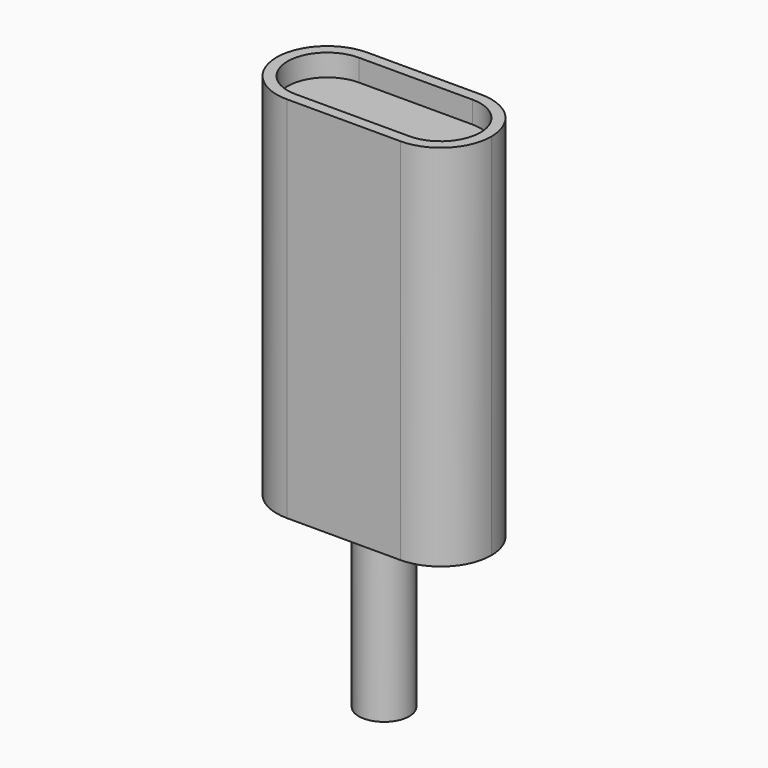
from build123d import *

# Parameters (mm, degrees)
F0_W     = 12.75
F0_H     = 6
F1_DEPTH = 21.9
F2_R     = 2.99999
F3_R     = 1.5
F4_DEPTH = 10
F6_DEPTH = 1.3


# Not quite as in the source:
# - a fillet or chamfer is up to 0.001 mm smaller than in the source, because OpenCascade refuses the exact size


with BuildPart() as f1:
    # F0 (on Top) → F1 (new body)
    with BuildSketch(Plane.XY):
        Rectangle(F0_W, F0_H)
    extrude(amount=F1_DEPTH)

    # F2 (radius 3 in the source; OpenCascade refuses exactly that, so slightly less here)
    f2_edges = [f1.edges().sort_by_distance(p)[0] for p in [
        (-6.375, -3, 10.95),
        (-6.375, 3, 10.95),
        (6.375, -3, 10.95),
        (6.375, 3, 10.95),
    ]]
    fillet(f2_edges, radius=F2_R)

    # F3 (on face) → F4 (join)
    with BuildSketch(Plane(origin=(0, 0, 0), x_dir=(1, 0, 0), z_dir=(0, 0, -1))):
        Circle(F3_R)
    extrude(amount=F4_DEPTH)

    # F5 (on face) → F6 (cut)
    with BuildSketch(Plane.XY.offset(21.9)):
        with BuildLine():
            Line((3.375, 2.35), (-3.375, 2.35))
            ThreePointArc((-3.375, 2.35), (-5.725, 0), (-3.375, -2.35))
            Line((-3.375, -2.35), (3.375, -2.35))
            ThreePointArc((3.375, -2.35), (5.725, 0), (3.375, 2.35))
        make_face()
    extrude(amount=-F6_DEPTH, mode=Mode.SUBTRACT)


solid = f1.part
